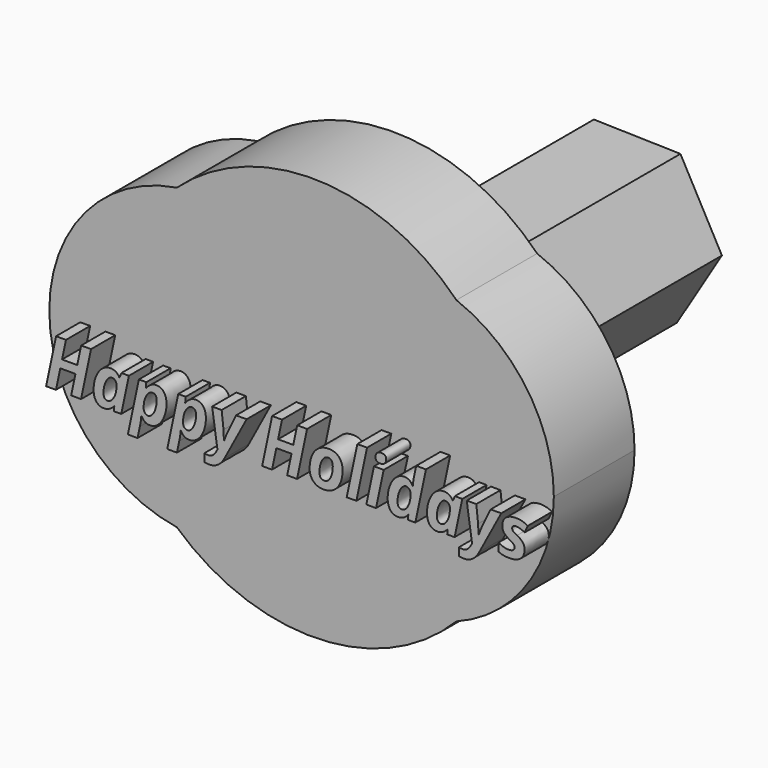
from build123d import *

# Parameters (mm, degrees)
F1_DEPTH     = 25.4
F3_DEPTH     = 76.2
F4_TEXT_SIZE = 16.6618744598
F5_DEPTH     = 7.62


# Not quite as in the source:
# - Text() gives the source's letters only with a copy of the font that has no kerning and outlines rounded to 1/6400 em; it was checked with that copy


with BuildPart() as f1:
    # F0 (on Front) → F1 (new body)
    with BuildSketch(Plane.XZ):
        with BuildLine():
            ThreePointArc((36.2430052256, -35.5961314221), (54.0370166652, -21.6108662323), (60.7589915411, 0))
            ThreePointArc((60.7589915411, 0), (54.0370166652, 21.6108662323), (36.2430052256, 35.5961314221))
            ThreePointArc((36.2430052256, 35.5961314221), (47.0201268898, 19.228823866), (50.8, 0))
            ThreePointArc((50.8, 0), (47.0201268898, -19.228823866), (36.2430052256, -35.5961314221))
        make_face()
        with BuildLine():
            ThreePointArc((-34.1307306007, -37.6262305934), (-50.8, 0), (-34.1307306007, 37.6262305934))
            ThreePointArc((-34.1307306007, 37.6262305934), (-66.2410084589, 0), (-34.1307306007, -37.6262305934))
        make_face()
        with BuildLine():
            ThreePointArc((-2.7410084589, 28.3980633142), (15.7410851184, 37.4666861455), (36.2430052256, 35.5961314221))
            ThreePointArc((36.2430052256, 35.5961314221), (1.4648384498, 50.7788760049), (-34.1307306007, 37.6262305934))
            ThreePointArc((-34.1307306007, 37.6262305934), (-17.3948701076, 36.5531190261), (-2.7410084589, 28.3980633142))
        make_face()
        with BuildLine():
            ThreePointArc((-34.1307306007, -37.6262305934), (1.4648384498, -50.7788760049), (36.2430052256, -35.5961314221))
            ThreePointArc((36.2430052256, -35.5961314221), (15.7410851184, -37.4666861455), (-2.7410084589, -28.3980633142))
            ThreePointArc((-2.7410084589, -28.3980633142), (-17.3948701076, -36.5531190261), (-34.1307306007, -37.6262305934))
        make_face()
        with BuildLine():
            ThreePointArc((50.8, 0), (47.0201268898, 19.228823866), (36.2430052256, 35.5961314221))
            ThreePointArc((36.2430052256, 35.5961314221), (15.7410851184, 37.4666861455), (-2.7410084589, 28.3980633142))
            ThreePointArc((-2.7410084589, 28.3980633142), (6.6393739427, 15.5542598667), (9.9589915411, 0))
            ThreePointArc((9.9589915411, 0), (6.6393739427, -15.5542598667), (-2.7410084589, -28.3980633142))
            ThreePointArc((-2.7410084589, -28.3980633142), (15.7410851184, -37.4666861455), (36.2430052256, -35.5961314221))
            ThreePointArc((36.2430052256, -35.5961314221), (47.0201268898, -19.228823866), (50.8, 0))
        make_face()
        with BuildLine():
            ThreePointArc((-2.7410084589, -28.3980633142), (-15.4410084589, 0), (-2.7410084589, 28.3980633142))
            ThreePointArc((-2.7410084589, 28.3980633142), (-17.3948701076, 36.5531190261), (-34.1307306007, 37.6262305934))
            ThreePointArc((-34.1307306007, 37.6262305934), (-50.8, 0), (-34.1307306007, -37.6262305934))
            ThreePointArc((-34.1307306007, -37.6262305934), (-17.3948701076, -36.5531190261), (-2.7410084589, -28.3980633142))
        make_face()
        with BuildLine():
            ThreePointArc((9.9589915411, 0), (6.6393739427, 15.5542598667), (-2.7410084589, 28.3980633142))
            ThreePointArc((-2.7410084589, 28.3980633142), (-15.4410084589, 0), (-2.7410084589, -28.3980633142))
            ThreePointArc((-2.7410084589, -28.3980633142), (6.6393739427, -15.5542598667), (9.9589915411, 0))
        make_face()
    extrude(amount=F1_DEPTH)

    # F2 (on face) → F3 (join)
    with BuildSketch(Plane(origin=(0, 0, 0), x_dir=(-1, 0, 0), z_dir=(0, 1, 0))):
        Polygon((21.7885982284, 0.5237985274), (10.440676283, 19.1313788423), (-11.3479219454, 18.6075803149), (-21.7885982284, -0.5237985274), (-10.440676283, -19.1313788423), (11.3479219454, -18.6075803149), align=None)
    extrude(amount=F3_DEPTH)

    # F4 (on face) → F5 (join)
    with BuildSketch(Plane.XZ.offset(25.4)):
        with Locations((-61.3820851682, -11.9965496111)):
            Text('Happy Holidays', F4_TEXT_SIZE, font='Open Sans', font_style=FontStyle.BOLDITALIC, text_align=(TextAlign.LEFT, TextAlign.BOTTOM))
    extrude(amount=F5_DEPTH)


solid = f1.part
